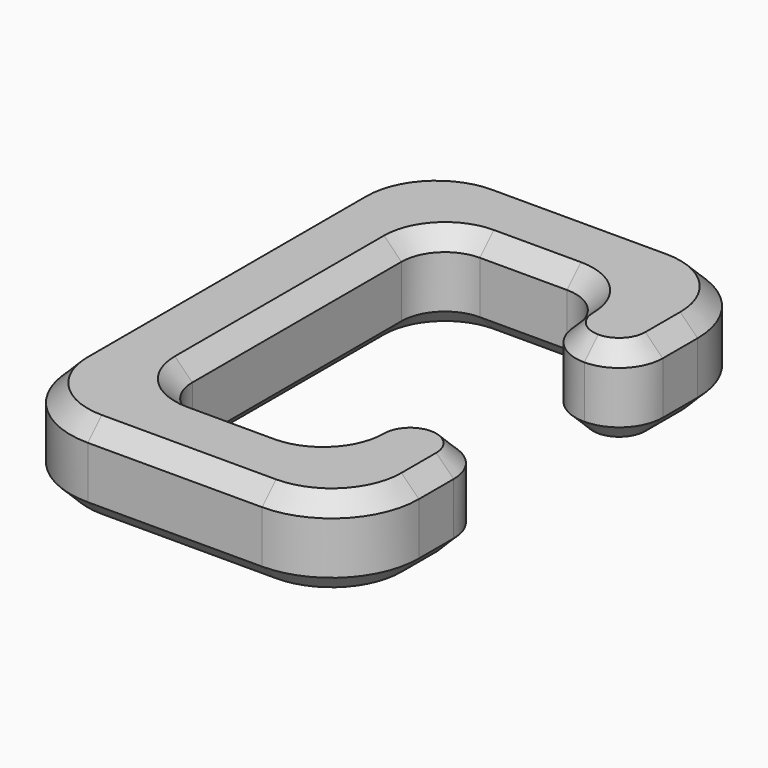
from build123d import *

# Parameters (mm, degrees)
F0_W     = 10
F0_H     = 10
F1_DEPTH = 10
F2_R     = 4.99999
F3_R     = 10
F4_SIZE  = 2


# Not quite as in the source:
# - a fillet or chamfer is up to 0.001 mm smaller than in the source, because OpenCascade refuses the exact size


with BuildPart() as f1:
    # F0 (on Top) → F1 (new body)
    with BuildSketch(Plane.XY):
        Polygon((6.4705845391, 30), (6.4705845391, 40), (-23.5294154609, 40), (-23.5294154609, 30), (-13.5294154609, 30), align=None)
        Polygon((16.4705845391, 40), (6.4705845391, 40), (6.4705845391, 30), (6.4705845391, 20), (16.4705845391, 20), align=None)
        Polygon((-13.5294154609, -10), (-13.5294154609, 30), (-23.5294154609, 30), (-23.5294154609, -20), (-13.5294154609, -20), align=None)
        Polygon((6.4705845391, -10), (-13.5294154609, -10), (-13.5294154609, -20), (16.4705845391, -20), (16.4705845391, -10), align=None)
        with Locations((11.4705845391, -5)):
            Rectangle(F0_W, F0_H)
    extrude(amount=F1_DEPTH)

    # F2 (radius 5 in the source; OpenCascade refuses exactly that, so slightly less here)
    f2_edges = [f1.edges().sort_by_distance(p)[0] for p in [
        (16.470585, 0, 5),
        (6.470585, 0, 5),
        (-13.529415, -10, 5),
        (6.470585, -10, 5),
        (6.470585, 20, 5),
        (6.470585, 30, 5),
        (-13.529415, 30, 5),
        (16.470585, 20, 5),
    ]]
    fillet(f2_edges, radius=F2_R)

    # F3
    f3_edges = [f1.edges().sort_by_distance(p)[0] for p in [
        (16.470585, 40, 5),
        (-23.529415, 40, 5),
        (16.470585, -20, 5),
        (-23.529415, -20, 5),
    ]]
    fillet(f3_edges, radius=F3_R)

    # F4
    f4_edges = [f1.edges().sort_by_distance(p)[0] for p in [
        (16.470585, 27.499995, 10),
        (13.541652, 37.071068, 10),
        (15.006121, 21.464463, 10),
        (-3.529415, 40, 10),
        (11.470585, 20, 10),
        (-20.600483, 37.071068, 10),
        (7.935048, 21.464463, 10),
        (-23.529415, 10, 10),
        (6.470585, 25, 10),
        (-20.600483, -17.071068, 10),
        (5.006121, 28.535537, 10),
        (-3.529415, -20, 10),
        (-3.529415, 30, 10),
        (13.541652, -17.071068, 10),
        (-12.064952, 28.535537, 10),
        (16.470585, -7.499995, 10),
        (-13.529415, 10, 10),
        (15.006121, -1.464463, 10),
        (-12.064952, -8.535537, 10),
        (11.470585, 0, 10),
        (-3.529415, -10, 10),
        (7.935048, -1.464463, 10),
        (5.006121, -8.535537, 10),
        (6.470585, -5, 10),
        (16.470585, 27.499995, 0),
        (13.541652, 37.071068, 0),
        (15.006121, 21.464463, 0),
        (-3.529415, 40, 0),
        (11.470585, 20, 0),
        (-20.600483, 37.071068, 0),
        (7.935048, 21.464463, 0),
        (-23.529415, 10, 0),
        (6.470585, 25, 0),
        (-20.600483, -17.071068, 0),
        (5.006121, 28.535537, 0),
        (-3.529415, -20, 0),
        (-3.529415, 30, 0),
        (13.541652, -17.071068, 0),
        (-12.064952, 28.535537, 0),
        (16.470585, -7.499995, 0),
        (-13.529415, 10, 0),
        (15.006121, -1.464463, 0),
        (-12.064952, -8.535537, 0),
        (11.470585, 0, 0),
        (-3.529415, -10, 0),
        (7.935048, -1.464463, 0),
        (5.006121, -8.535537, 0),
        (6.470585, -5, 0),
    ]]
    chamfer(f4_edges, length=F4_SIZE)


solid = f1.part
